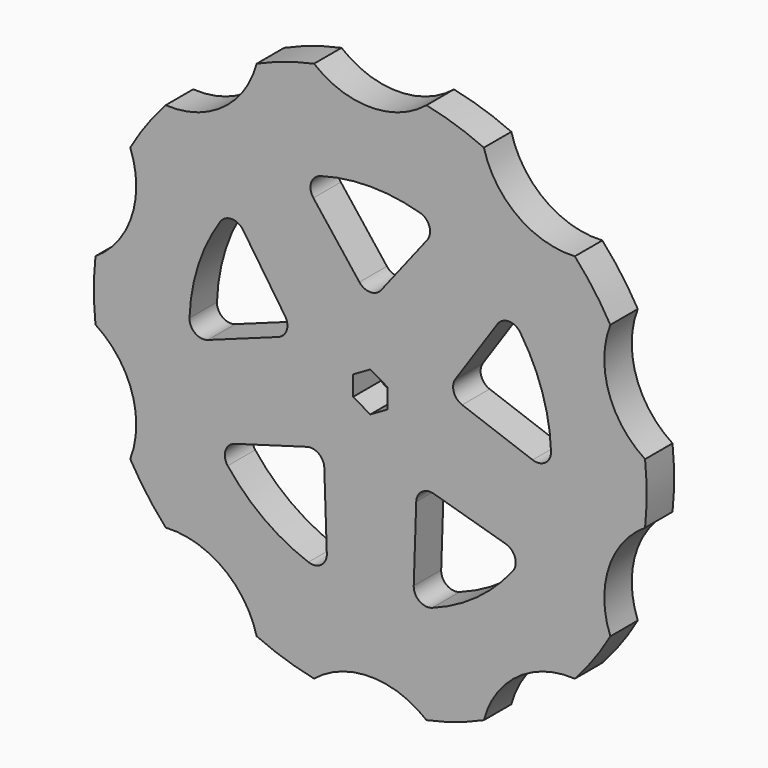
from build123d import *

# Parameters (mm, degrees)
F0_R            = 51.1347366711
F4_DEPTH        = 3.175
F2_R            = 16.4453954174
F5_DEPTH        = 12.7
F6_DEPTH        = 12.7
F7_DEPTH        = 12.7
F7_COPIES_COUNT = 5


# Not quite as in the source:
# - a pattern or mirror of a feature is missing from the dataset's text; its kind, count and spacing are read off the source's solid


with BuildPart() as f4:
    # F0 (on Front) → F4 (new body, symmetric)
    with BuildSketch(Plane.XZ):
        Circle(F0_R)
    extrude(amount=F4_DEPTH, both=True)

    # F2 (on Front) → F5 (cut, symmetric)
    with BuildSketch(Plane.XZ):
        with Locations((0, 62.8050640225)):
            Circle(F2_R)
        with Locations((36.9158904017, 50.810364127)):
            Circle(F2_R)
        with Locations((-36.9158904017, 50.810364127)):
            Circle(F2_R)
        with Locations((-59.731165395, 19.4078321158)):
            Circle(F2_R)
        with Locations((-59.731165395, -19.4078321158)):
            Circle(F2_R)
        with Locations((-36.9158904017, -50.810364127)):
            Circle(F2_R)
        with Locations((0, -62.8050640225)):
            Circle(F2_R)
        with Locations((36.9158904017, -50.810364127)):
            Circle(F2_R)
        with Locations((59.731165395, -19.4078321158)):
            Circle(F2_R)
        with Locations((59.731165395, 19.4078321158)):
            Circle(F2_R)
    extrude(amount=F5_DEPTH, both=True, mode=Mode.SUBTRACT)

    # F1 (on Front) → F6 (cut, symmetric)
    with BuildSketch(Plane.XZ):
        Polygon((0.0026473821, -3.6661732535), (3.1763228633, -1.8307939266), (3.1736754811, 1.8353793269), (-0.0026473821, 3.6661732535), (-3.1763228633, 1.8307939266), (-3.1736754811, -1.8353793269), align=None)
    extrude(amount=F6_DEPTH, both=True, mode=Mode.SUBTRACT)

    # F3 (on Front) → F7 (cut, symmetric)
    with BuildSketch(Plane.XZ):
        with BuildLine():
            Line((2.0035802963, 17.2253447383), (10.5229329015, 28.1589119968))
            ThreePointArc((10.5229329015, 28.1589119968), (10.9344914514, 30.5066641744), (9.2192630979, 32.1617510067))
            ThreePointArc((9.2192630979, 32.1617510067), (0, 33.4570327418), (-9.2192630979, 32.1617510067))
            ThreePointArc((-9.2192630979, 32.1617510067), (-10.9344914514, 30.5066641744), (-10.5229329015, 28.1589119968))
            Line((-10.5229329015, 28.1589119968), (-2.0035802963, 17.2253447383))
            ThreePointArc((-2.0035802963, 17.2253447383), (0, 16.246519295), (2.0035802963, 17.2253447383))
        make_face()
    f7 = extrude(amount=F7_DEPTH, both=True, mode=Mode.SUBTRACT)

    # F7_copies: F7 ×5 about axis
    f7_copies_axis = Axis((0, 0, 0), (0, 1, 0))
    for i in range(1, F7_COPIES_COUNT):
        add(f7.rotate(f7_copies_axis, i * 360 / F7_COPIES_COUNT), mode=Mode.SUBTRACT)


solid = f4.part
